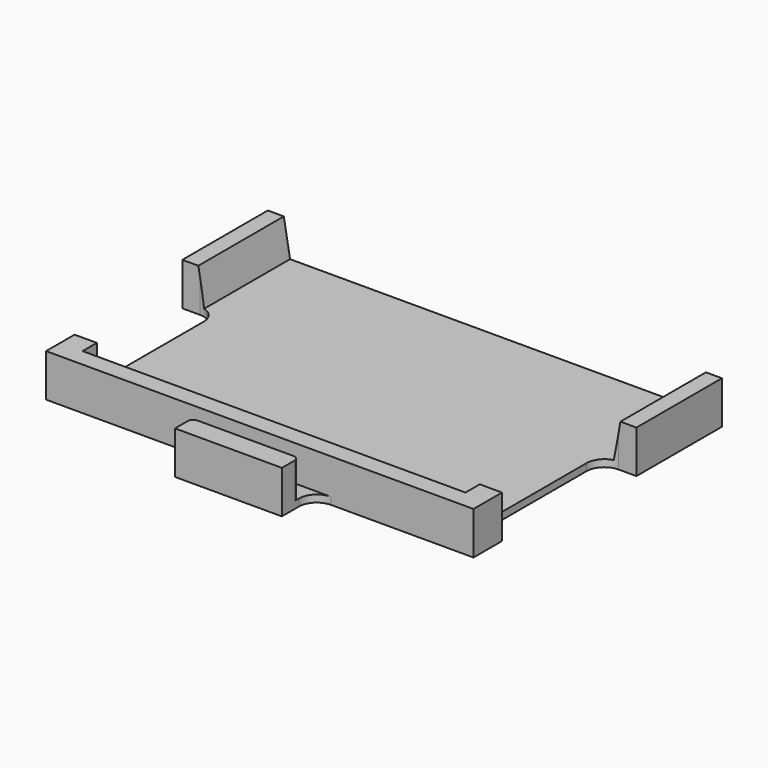
from build123d import *

# Parameters (mm, degrees)
F0_W     = 6
F0_H     = 1
F0_H_2   = 1.2
F0_W_2   = 1.1
F0_H_3   = 6
F0_W_3   = 0.9
F5_DEPTH = 6
F6_R     = 1
F7_R     = 0.3


with BuildPart() as f2:
    # F2: sweep along a path in F1
    with BuildLine(Plane.XZ) as f2_path:
        Line((0, 0), (0, 0.4))
    # F0 (on Top) → F2 (sweep)
    with BuildSketch(Plane.XY):
        Polygon((-10.75, 1), (-10.75, 0), (-3, 0), (3, 0), (10.75, 0), (10.75, 1), align=None)
        Polygon((-12, 0), (-10.75, 0), (-10.75, 1), (-10.75, 2), (-12, 2), align=None)
        with Locations((0, -0.5)):
            Rectangle(F0_W, F0_H)
        Polygon((-10.75, 2), (-10.75, 1), (10.75, 1), (10.75, 2), (10.75, 10.5), (10.75, 16.5), (-10.75, 16.5), (-10.75, 10.5), align=None)
        with Locations((0, -1.6)):
            Rectangle(F0_W, F0_H_2)
        Polygon((10.75, 2), (10.75, 1), (10.75, 0), (12, 0), (12, 2), align=None)
        with Locations((-11.3, 13.5)):
            Rectangle(F0_W_2, F0_H_3)
        with Locations((-12.3, 13.5)):
            Rectangle(F0_W_3, F0_H_3)
        with Locations((11.3, 13.5)):
            Rectangle(F0_W_2, F0_H_3)
        with Locations((12.3, 13.5)):
            Rectangle(F0_W_3, F0_H_3)
    sweep(path=f2_path.line)

    # F3: sweep along a path in F1
    with BuildLine(Plane.XZ) as f3_path:
        Line((0, 0), (0, 0.4))
        Line((0, 0.4), (0, 2.4))
    # F0 (on Top) → F3 (sweep)
    with BuildSketch(Plane.XY):
        Polygon((-10.75, 1), (-10.75, 0), (-3, 0), (3, 0), (10.75, 0), (10.75, 1), align=None)
        Polygon((-12, 0), (-10.75, 0), (-10.75, 1), (-10.75, 2), (-12, 2), align=None)
        Polygon((10.75, 2), (10.75, 1), (10.75, 0), (12, 0), (12, 2), align=None)
        with Locations((12.3, 13.5)):
            Rectangle(F0_W_3, F0_H_3)
        with Locations((-12.3, 13.5)):
            Rectangle(F0_W_3, F0_H_3)
        with Locations((0, -1.6)):
            Rectangle(F0_W, F0_H_2)
    sweep(path=f3_path.line)

    # F4 (on face) → F5 (join, through all)
    with BuildSketch(Plane(origin=(0, 16.5, 0), x_dir=(-1, 0, 0), z_dir=(0, 1, 0))):
        Polygon((-11.5, 0.4), (-11.85, 2.4), (-11.85, 0.4), align=None)
        Polygon((11.85, 2.4), (11.5, 0.4), (11.85, 0.4), align=None)
    extrude(amount=-F5_DEPTH)

    # F6
    f6_edges = [f2.edges().sort_by_distance(p)[0] for p in [
        (-10.75, 10.5, 0.2),
        (10.75, 10.5, 0.2),
        (3, 0, 0.2),
        (-3, 0, 0.2),
    ]]
    fillet(f6_edges, radius=F6_R)

    # F7
    f7_edges = [f2.edges().sort_by_distance(p)[0] for p in [
        (-3, -1, 1.4),
        (3, -1, 1.4),
    ]]
    fillet(f7_edges, radius=F7_R)


solid = f2.part
